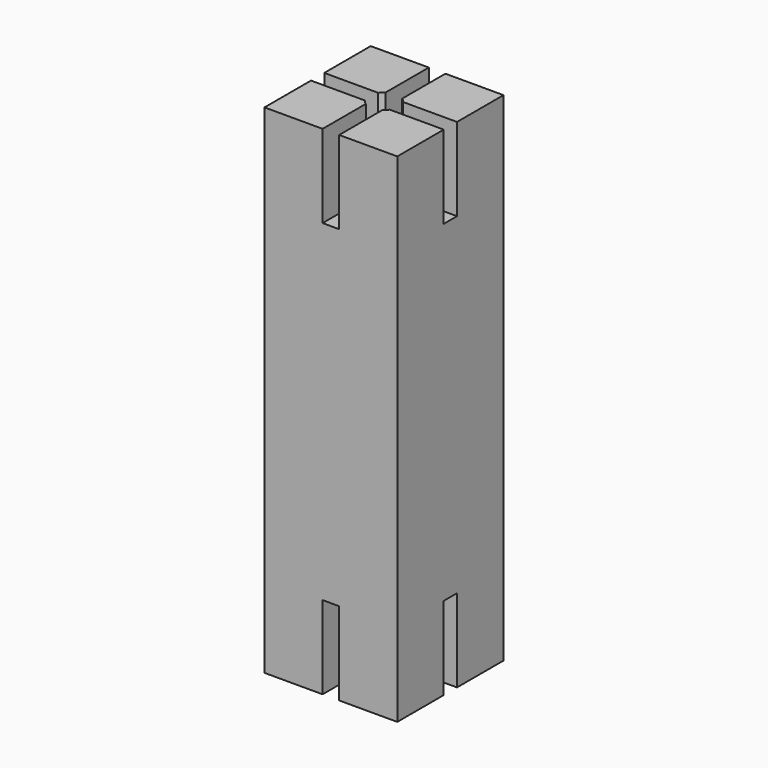
from build123d import *

# Parameters (mm, degrees)
F0_W          = 8
F0_H          = 8
F1_DEPTH      = 15
F1_DEPTH_BACK = 15
F2_R          = 0.9
F3_DEPTH      = 36.9
F4_W          = 4.5
F4_H          = 1
F4_W_2        = 1
F4_H_2        = 4.5
F5_DEPTH      = 5


# Not quite as in the source:
# - a pattern or mirror of a feature is missing from the dataset's text; its kind, count and spacing are read off the source's solid


with BuildPart() as f1:
    # F0 (on Top) → F1 (new body, two sides)
    with BuildSketch(Plane.XY) as f1_sk:
        Rectangle(F0_W, F0_H)
    extrude(amount=F1_DEPTH)
    extrude(f1_sk.sketch, amount=-F1_DEPTH_BACK)

    # F2 (on face) → F3 (cut)
    with BuildSketch(Plane.XY.offset(15)):
        Circle(F2_R)
    extrude(amount=-F3_DEPTH, mode=Mode.SUBTRACT)

    # F4 (on face) → F5 (cut)
    with BuildSketch(Plane.XY.offset(15)):
        with Locations((-2.75, 0)):
            Rectangle(F4_W, F4_H)
        Rectangle(F4_W_2, F4_H)
        with Locations((0, -2.75)):
            Rectangle(F4_W_2, F4_H_2)
        with Locations((2.75, 0)):
            Rectangle(F4_W, F4_H)
        with Locations((0, 2.75)):
            Rectangle(F4_W_2, F4_H_2)
    f5 = extrude(amount=-F5_DEPTH, mode=Mode.SUBTRACT)

    # F5_copies: F5 across plane
    add(f5.mirror(Plane(origin=(0, 0, 0), x_dir=(-1, 0, 0), z_dir=(0, 0, -1))), mode=Mode.SUBTRACT)


solid = f1.part
